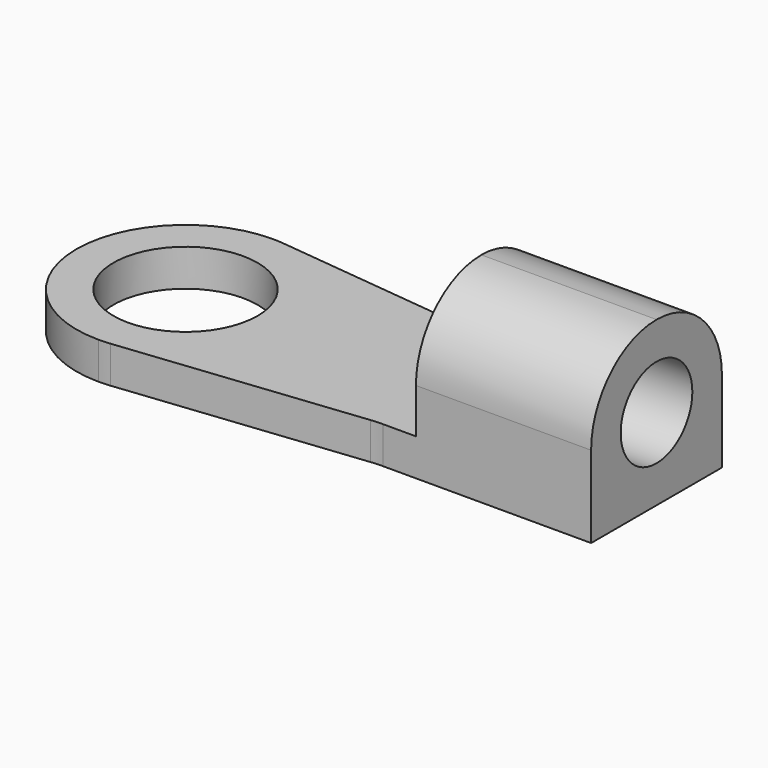
from build123d import *

# Parameters (mm, degrees)
F0_R     = 1.85
F1_DEPTH = 0.95
F2_W     = 4.5
F2_H     = 4.2
F3_DEPTH = 3.25
F4_R     = 2.09999
F5_R     = 1.15
F6_DEPTH = 25


# Not quite as in the source:
# - a fillet or chamfer is up to 0.001 mm smaller than in the source, because OpenCascade refuses the exact size


with BuildPart() as f1:
    # F0 (on Top) → F1 (new body)
    with BuildSketch(Plane.XY):
        with BuildLine():
            Line((9.5515289224, 0.7), (14.9, 0.7))
            Line((14.9, 0.7), (14.9, 4.9))
            Line((14.9, 4.9), (10.4, 4.9))
            Line((10.4, 4.9), (9.5515289224, 4.9))
            ThreePointArc((9.5515289224, 4.9), (9.4002214052, 4.9040911969), (9.2493560516, 4.916352832))
            Line((9.2493560516, 4.916352832), (3.1021728708, 5.583647168))
            ThreePointArc((3.1021728708, 5.583647168), (2.9513075171, 5.5959088031), (2.8, 5.6))
            ThreePointArc((2.8, 5.6), (0.8201010127, 4.7798989873), (0, 2.8))
            ThreePointArc((0, 2.8), (0.8201010127, 0.8201010127), (2.8, 0))
            ThreePointArc((2.8, 0), (2.9513075171, 0.0040911969), (3.1021728708, 0.016352832))
            Line((3.1021728708, 0.016352832), (9.2493560516, 0.683647168))
            ThreePointArc((9.2493560516, 0.683647168), (9.4002214052, 0.6959088031), (9.5515289224, 0.7))
        make_face()
        with Locations((2.8, 2.8)):
            Circle(F0_R, mode=Mode.SUBTRACT)
    extrude(amount=F1_DEPTH)

    # F2 (on face) → F3 (join)
    with BuildSketch(Plane.XY.offset(0.95)):
        with Locations((12.65, 2.8)):
            Rectangle(F2_W, F2_H)
    extrude(amount=F3_DEPTH)

    # F4 (radius 2.1 in the source; OpenCascade refuses exactly that, so slightly less here)
    f4_edges = [f1.edges().sort_by_distance(p)[0] for p in [
        (12.65, 4.9, 4.2),
        (12.65, 0.7, 4.2),
    ]]
    fillet(f4_edges, radius=F4_R)

    # F5 (on face) → F6 (cut)
    with BuildSketch(Plane.YZ.offset(14.9)):
        with Locations((2.8, 2.1)):
            Circle(F5_R)
    extrude(amount=-F6_DEPTH, mode=Mode.SUBTRACT)


solid = f1.part
